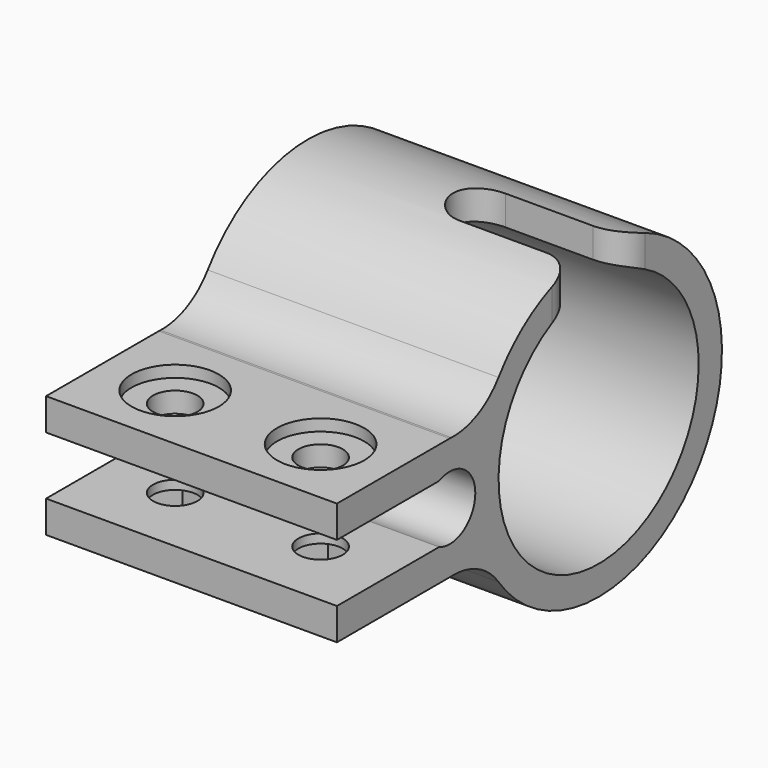
from build123d import *

# Parameters (mm, degrees)
F1_DEPTH  = 25
F3_DEPTH  = 3.96875
F4_R      = 3.81
F5_DEPTH  = 21.001
F6_R      = 7.5
F7_DEPTH  = 2
F8_R      = 26.5
F8_R_2    = 21.5
F9_DEPTH  = 25
F10_W     = 41.7897145033
F10_H     = 10
F11_DEPTH = 26.501
F12_R     = 5
F13_R     = 12


# Not quite as in the source:
# - a length typed as a fraction of an inch, garbled in the dataset ("3 / 203.2 mm" for 3/8 in), is restored


with BuildPart() as f1:
    # F0 (on Right) → F1 (new body, symmetric)
    with BuildSketch(Plane.YZ):
        with BuildLine():
            Line((-24.2330926563, 5), (-9.2330926563, 5))
            ThreePointArc((-9.2330926563, 5), (-5.3735463151, 9.0208092763), (0, 10.5))
            Line((0, 10.5), (-24.2330926563, 10.5))
            Line((-24.2330926563, 10.5), (-24.2330926563, 5))
        make_face()
        with BuildLine():
            ThreePointArc((-2.2912878475, 5), (2.9705148408, 4.628827236), (5.5, 0))
            ThreePointArc((5.5, 0), (2.9705148408, -4.628827236), (-2.2912878475, -5))
            Line((-2.2912878475, -5), (-9.2330926563, -5))
            ThreePointArc((-9.2330926563, -5), (-5.3735463151, -9.0208092763), (0, -10.5))
            ThreePointArc((0, -10.5), (7.4246212025, -7.4246212025), (10.5, 0))
            ThreePointArc((10.5, 0), (7.4246212025, 7.4246212025), (0, 10.5))
            ThreePointArc((0, 10.5), (-5.3735463151, 9.0208092763), (-9.2330926563, 5))
            Line((-9.2330926563, 5), (-2.2912878475, 5))
        make_face()
        with BuildLine():
            ThreePointArc((0, -10.5), (-5.3735463151, -9.0208092763), (-9.2330926563, -5))
            Line((-9.2330926563, -5), (-24.2330926563, -5))
            Line((-24.2330926563, -5), (-24.2330926563, -10.5))
            Line((-24.2330926563, -10.5), (0, -10.5))
        make_face()
    extrude(amount=F1_DEPTH, both=True)

    # F2 (on face) → F3 (cut)
    with BuildSketch(Plane(origin=(0, 0, -10.5), x_dir=(1, 0, 0), z_dir=(0, 0, -1))):
        Polygon((19.1395280957, 12.1165463282), (15.8197640478, 17.8665463282), (9.1802359522, 17.8665463282), (5.8604719043, 12.1165463282), (9.1802359522, 6.3665463282), (15.8197640478, 6.3665463282), align=None)
        Polygon((-15.8197640478, 6.3665463282), (-9.1802359522, 6.3665463282), (-5.8604719043, 12.1165463282), (-9.1802359522, 17.8665463282), (-15.8197640478, 17.8665463282), (-19.1395280957, 12.1165463282), align=None)
    extrude(amount=-F3_DEPTH, mode=Mode.SUBTRACT)

    # F4 (on face) → F5 (cut, through all)
    with BuildSketch(Plane(origin=(0, 0, -10.5), x_dir=(1, 0, 0), z_dir=(0, 0, -1))):
        with Locations((12.5, 12.1165463282)):
            Circle(F4_R)
        with Locations((-12.5, 12.1165463282)):
            Circle(F4_R)
    extrude(amount=-F5_DEPTH, mode=Mode.SUBTRACT)

    # F6 (on face) → F7 (cut)
    with BuildSketch(Plane.XY.offset(10.5)):
        with Locations((-12.5, -12.1165463282)):
            Circle(F6_R)
        with Locations((12.5, -12.1165463282)):
            Circle(F6_R)
    extrude(amount=-F7_DEPTH, mode=Mode.SUBTRACT)

    # F8 (on Right) → F9 (join, symmetric)
    with BuildSketch(Plane.YZ):
        with Locations((32, 0)):
            Circle(F8_R)
        with Locations((32, 0)):
            Circle(F8_R_2, mode=Mode.SUBTRACT)
    extrude(amount=F9_DEPTH, both=True)

    # F10 (on Top) → F11 (cut, through all)
    with BuildSketch(Plane.XY):
        with Locations((25.8948572517, 32)):
            Rectangle(F10_W, F10_H)
        with BuildLine():
            ThreePointArc((5, 37), (0, 32), (5, 27))
            Line((5, 27), (5, 37))
        make_face()
    extrude(amount=F11_DEPTH, mode=Mode.SUBTRACT)

    # F12
    f12_edges = [f1.edges().sort_by_distance(p)[0] for p in [
        (25, 27, 23.467276),
        (25, 37, 23.467276),
    ]]
    fillet(f12_edges, radius=F12_R)

    # F13
    f13_edges = [f1.edges().sort_by_distance(p)[0] for p in [
        (0, 6.75, 8.042854),
        (0, 6.75, -8.042854),
    ]]
    fillet(f13_edges, radius=F13_R)


solid = f1.part
